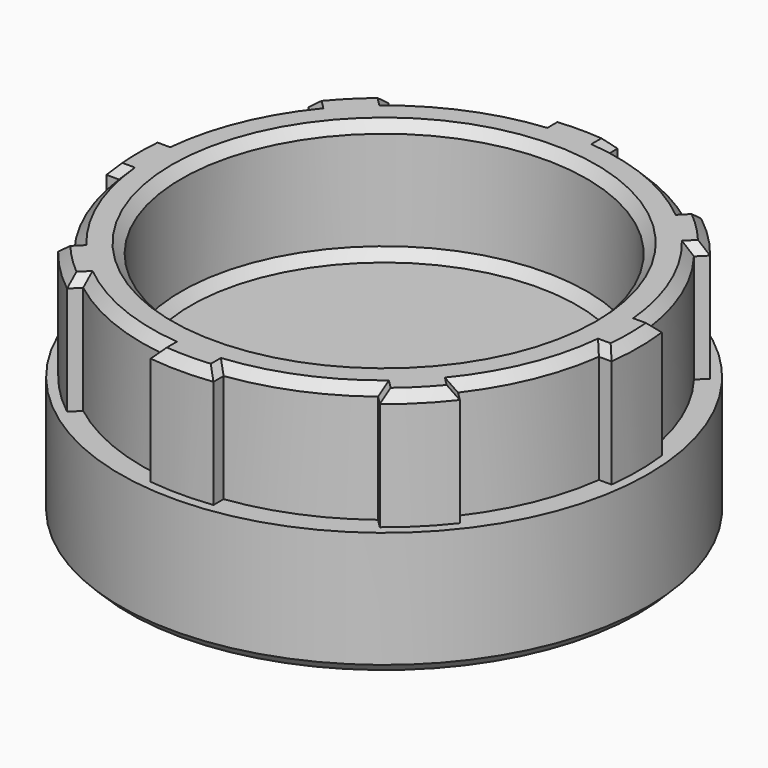
from build123d import *

# Parameters (mm, degrees)
F0_R            = 8.4
F1_DEPTH        = 4
F2_R            = 7.7
F2_R_2          = 6.45
F3_DEPTH        = 3.75
F5_DEPTH        = 3.75
F5_COPIES_COUNT = 8
F7_SIZE         = 0.3


# Not quite as in the source:
# - a pattern or mirror of a feature is missing from the dataset's text; its kind, count and spacing are read off the source's solid


with BuildPart() as f1:
    # F0 (on Top) → F1 (new body)
    with BuildSketch(Plane.XY):
        Circle(F0_R)
    extrude(amount=F1_DEPTH)

    # F2 (on face) → F3 (join)
    with BuildSketch(Plane.XY.offset(4)):
        Circle(F2_R)
        Circle(F2_R_2, mode=Mode.SUBTRACT)
    extrude(amount=F3_DEPTH)

    # F4 (on face) → F5 (join, through all)
    with BuildSketch(Plane.XY.offset(4)):
        with BuildLine():
            Line((1, 7.6347887987), (1, 8.0380345856))
            ThreePointArc((1, 8.0380345856), (0, 8.1), (-1, 8.0380345856))
            Line((-1, 8.0380345856), (-1, 7.6347887987))
            ThreePointArc((-1, 7.6347887987), (0, 7.7), (1, 7.6347887987))
        make_face()
    f5 = extrude(amount=F5_DEPTH)

    # F5_copies: F5 ×8 about axis
    f5_copies_axis = Axis((0, 0, 0), (0, 0, 1))
    for i in range(1, F5_COPIES_COUNT):
        add(f5.rotate(f5_copies_axis, i * 360 / F5_COPIES_COUNT))

    # F7
    f7_edges = [f1.edges().sort_by_distance(p)[0] for p in [
        (-8.4, 0, 0),
        (-6.45, 0, 4),
        (1, 7.836412, 7.75),
        (0, 8.1, 7.75),
        (-1, 7.836412, 7.75),
        (-2.946662, 7.113872, 7.75),
        (-4.834073, 6.248287, 7.75),
        (-5.727565, 5.727565, 7.75),
        (-6.248287, 4.834073, 7.75),
        (-7.113872, 2.946662, 7.75),
        (-7.836412, 1, 7.75),
        (-8.1, 0, 7.75),
        (-7.836412, -1, 7.75),
        (-7.113872, -2.946662, 7.75),
        (-6.248287, -4.834073, 7.75),
        (-5.727565, -5.727565, 7.75),
        (-4.834073, -6.248287, 7.75),
        (-2.946662, -7.113872, 7.75),
        (-1, -7.836412, 7.75),
        (0, -8.1, 7.75),
        (1, -7.836412, 7.75),
        (2.946662, -7.113872, 7.75),
        (4.834073, -6.248287, 7.75),
        (5.727565, -5.727565, 7.75),
        (6.248287, -4.834073, 7.75),
        (7.113872, -2.946662, 7.75),
        (7.836412, -1, 7.75),
        (8.1, 0, 7.75),
        (7.836412, 1, 7.75),
        (7.113872, 2.946662, 7.75),
        (6.248287, 4.834073, 7.75),
        (5.727565, 5.727565, 7.75),
        (4.834073, 6.248287, 7.75),
        (2.946662, 7.113872, 7.75),
        (-6.45, 0, 7.75),
    ]]
    chamfer(f7_edges, length=F7_SIZE)


solid = f1.part
